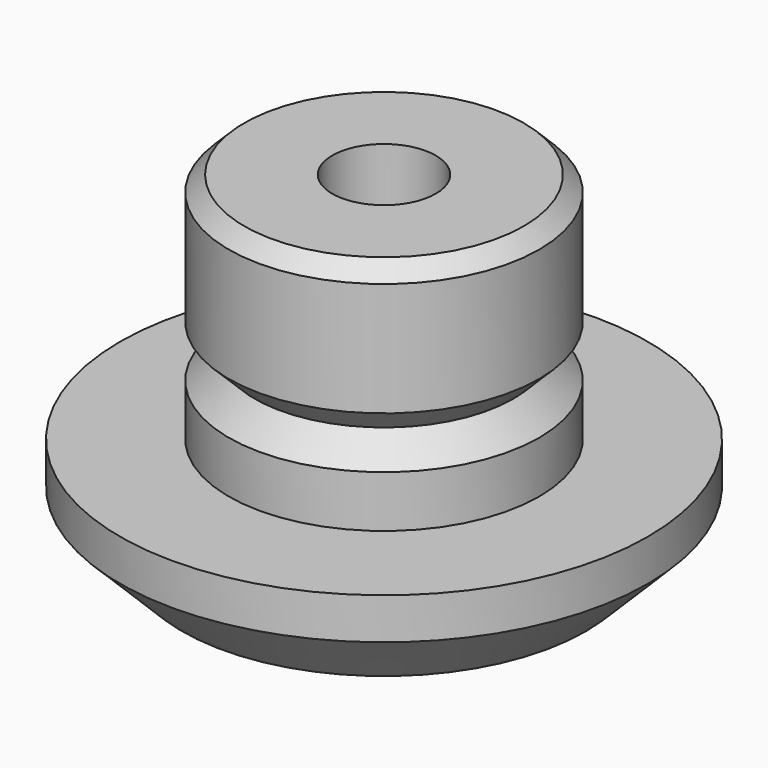
from build123d import *

# Parameters (mm, degrees)
F2_SIZE = 0.3
F3_SIZE = 0.49999
F4_SIZE = 1.2


# Not quite as in the source:
# - a fillet or chamfer is up to 0.001 mm smaller than in the source, because OpenCascade refuses the exact size


with BuildPart() as f1:
    # F0 (on Front) → F1 (revolve)
    with BuildSketch(Plane.XZ):
        Polygon((5.1, -2), (5.1, 0), (3, 0), (3, 1), (2.5, 1), (2.5, 2), (3, 2), (3, 4.5), (1, 4.5), (1, 2), (0, 2), (0, 0), (0, -2), align=None)
    revolve(axis=Axis((0, 0, -1), (0, 0, -1)))

    # F2
    f2_edges = [f1.edges().sort_by_distance(p)[0] for p in [
        (-3, 0, 4.5),
    ]]
    chamfer(f2_edges, length=F2_SIZE)

    # F3 (size 0.5 in the source; OpenCascade refuses exactly that, so slightly less here)
    f3_edges = [f1.edges().sort_by_distance(p)[0] for p in [
        (-2.5, 0, 2),
        (-2.5, 0, 1),
    ]]
    chamfer(f3_edges, length=F3_SIZE)

    # F4
    f4_edges = [f1.edges().sort_by_distance(p)[0] for p in [
        (-5.1, 0, -2),
    ]]
    chamfer(f4_edges, length=F4_SIZE)


solid = f1.part
